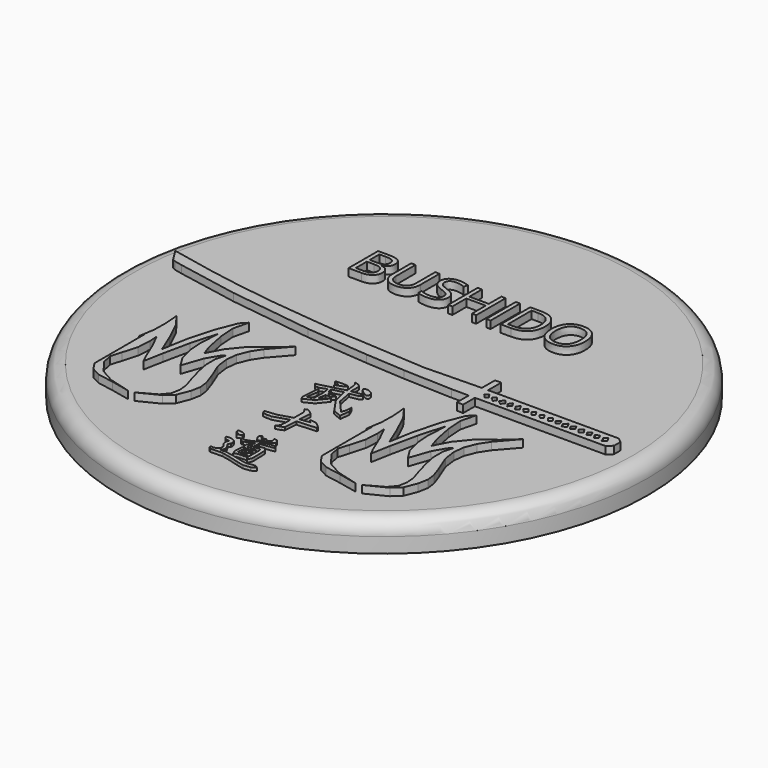
from build123d import *

# Parameters (mm, degrees)
F0_R         = 44.6165868488
F1_DEPTH     = 5.08
F2_R         = 2.54
F3_TEXT_SIZE = 8.7433378212
F4_DEPTH     = 1.27
F6_DEPTH     = 0.508
F8_DEPTH     = 1.27
F12_DEPTH    = 1.27


# Not quite as in the source:
# - Text() gives the source's letters only with a copy of the font that has no kerning and outlines rounded to 1/6400 em; it was checked with that copy


with BuildPart() as f1:
    # F0 (on Top) → F1 (new body)
    with BuildSketch(Plane.XY):
        with Locations((38.1, 0)):
            Circle(F0_R)
    extrude(amount=-F1_DEPTH)

    # F2
    f2_edges = [f1.edges().sort_by_distance(p)[0] for p in [
        (-6.516587, 0, 0),
    ]]
    fillet(f2_edges, radius=F2_R)

    # F3 (on Top) → F4 (join)
    with BuildSketch(Plane.XY):
        with Locations((18.0598776788, 16.4687121287)):
            Text('BUSHIDO', F3_TEXT_SIZE, font='Open Sans', text_align=(TextAlign.LEFT, TextAlign.BOTTOM))
    extrude(amount=F4_DEPTH)

    # F5 (on Top) → F6 (join)
    with BuildSketch(Plane.XY):
        with BuildLine():
            add(Edge.make_bspline(
                [(36.8690937757, -8.8045168668), (36.9262235113, -8.6325223752), (40.9652755864, -8.523144564), (36.521565131, -9.9590094355), (38.386831886, -9.2135998908), (36.830176095, -8.9216822386), (36.8690937757, -8.8045168668)],
                knots=[0, 0, 0, 0, 0.323818666, 0.6224903435, 0.7794095959, 1, 1, 1, 1], degree=3))
        make_face()
        with BuildLine():
            add(Edge.make_bspline(
                [(41.1289557815, -8.1255994737), (41.052845758, -8.4618202993), (42.8844335846, -10.000238978), (42.9689741831, -8.112585225), (41.197261541, -7.8238544756), (41.1289557815, -8.1255994737)],
                knots=[0, 0, 0, 0, 0.3876451352, 0.6521037019, 1, 1, 1, 1], degree=3))
        make_face()
        Polygon((39.8083478212, -7.551421877), (39.1193367541, -7.3983082548), (39.4829809666, -7.9342070967), (39.6935120225, -9.8098535091), (35.9422191978, -10.7859550044), (35.1766496897, -10.9582077712), (35.6551297009, -11.4941066131), (36.4207029343, -11.4941066131), (37.4733582139, -11.0730435699), (37.645611912, -12.2596770525), (37.645611912, -14.173601754), (36.6503708065, -14.556386508), (36.9566008449, -12.8338541836), (36.8226245046, -12.2788157314), (36.4207029343, -11.8194743991), (36.4207029343, -12.3745119199), (36.2527528205, -14.2884366214), (36.2527528205, -14.9953767122), (36.4589802921, -15.4176522046), (38.104955107, -14.6138044074), (39.4829809666, -12.9104116932), (38.8896651566, -13.4080322459), (38.104955107, -13.7716773897), (38.3154861629, -12.6233221963), (39.2150320113, -12.6233221963), (39.5786762238, -12.0108667761), (39.0427783132, -12.0108667761), (38.3537635207, -12.2213987634), (38.3537635207, -11.8768922985), (37.9712446996, -11.4986467292), (37.8296082923, -10.9278071133), (39.712652564, -10.4605872184), (40.3442457318, -13.0061078817), (42.0093610883, -15.4176522046), (43.4830822051, -16.0109698772), (43.6936169863, -14.3267158419), (43.2151332498, -13.2549181581), (43.2151332498, -14.2118800431), (42.8897663951, -15.09228535), (40.9145871592, -12.8176152195), (40.4590815306, -10.3648910299), (41.7988300323, -10.1160807535), (42.3921458423, -9.7907138988), (41.9136658311, -9.427068755), (40.2485504746, -9.7141573206), (40.2485504746, -7.9916249961), align=None)
        Polygon((39.1193367541, -17.3568017781), (38.6665798724, -17.5016503781), (39.1193367541, -18.2741675526), (39.1193367541, -20.3020274639), (36.7674715817, -21.0101678967), (34.7878970206, -21.2193913758), (35.0510981124, -21.753220402), (35.6730744243, -21.8309685588), (36.574345082, -21.8309685588), (39.1006264007, -21.0423562676), (39.1006264007, -22.0924360227), (38.9723666012, -23.1184996665), (38.521733135, -23.5852282494), (39.4069105387, -23.3277231455), (39.8092642426, -23.0863112956), (39.9702042341, -20.8814162761), (43.2695001364, -20.6721927971), (43.2695001364, -20.4307809472), (42.3491622125, -19.6015631681), (41.1289818585, -19.449038431), (41.4846295613, -19.8708384333), (41.6761822999, -19.9479572475), (39.95411098, -20.1893690974), (40.0989577174, -18.0488489568), (39.4835314239, -17.5034259469), align=None)
        Polygon((36.465685972, -27.7904520939), (35.5846919119, -27.6803262532), (35.6803871691, -28.1205289066), (36.2975304264, -28.466149787), (36.1146872415, -28.5084608213), (36.1397303641, -28.7234149873), (36.914074972, -28.4093043748), (36.809604615, -27.9578454792), align=None)
        Polygon((39.1804466829, -27.2458239053), (39.1193367541, -26.9817430526), (38.8000831008, -27.1731354296), (38.8000831008, -27.5463499129), (39.0297546983, -27.9961228371), (39.5869397098, -28.3664732433), (40.0249958038, -27.2784009576), (39.4795276225, -27.6229083538), align=None)
        Polygon((41.3673612083, -26.7059249962), (40.9101359546, -26.6487710178), (40.9225635231, -26.6326684505), (40.8548973501, -26.7138704658), (40.9015711261, -26.9170331416), (40.9766957164, -27.2416770458), (40.0902554393, -28.1890202314), (39.0414074063, -28.9130620658), (38.0263961852, -29.2311012745), (37.4647565186, -29.2311012745), (37.4985933304, -29.4950027019), (37.7286598086, -29.7453738749), (38.1211340427, -29.7859739512), (39.7722199559, -29.1498992592), (38.9661676253, -30.252532206), (39.1075549029, -30.6578476496), (39.0109978616, -31.4302928746), (38.9168218354, -32.5174966777), (39.1666330397, -33.2336314023), (39.5207442189, -33.0261609126), (40.0767624378, -32.9613823011), (40.8199538526, -32.9613823011), (41.1932729185, -32.8749939799), (41.2406399846, -32.766725868), (41.0883910954, -32.4960537255), (40.7293175893, -32.4298856209), (40.0632284582, -32.5840227306), (39.6606065333, -32.5366556644), (39.684291929, -32.4723720551), (39.3933206797, -32.5907878578), (39.4289206542, -31.9954107358), (39.500977844, -31.8164303899), (40.4062718153, -31.8928770721), (40.1003203773, -32.2016964793), (40.1447415352, -32.2630405426), (40.4947884381, -32.0095606148), (41.0145658499, -31.7668251122), (41.1063656211, -31.5388068557), (40.9172587097, -31.3875525708), (40.5635686484, -31.3875525708), (39.875164628, -31.5468534827), (39.4526943564, -31.5508767962), (39.4526943564, -31.0439113528), (39.9654139058, -31.0475337206), (40.07634148, -31.0921929777), (39.8872345686, -31.2531366944), (39.9556346238, -31.3014164567), (40.2260981022, -31.1137784975), (40.7724119723, -30.9232063591), (40.9937053919, -30.7019110769), (40.8166721463, -30.5288992822), (40.5430719256, -30.508780852), (40.0766329326, -30.6154663914), (39.5159046677, -30.6942713389), (39.4848845899, -30.6053459644), (39.3802709877, -30.2150640637), (39.6498478949, -30.0380289555), (40.0692522526, -30.0380289555), (40.7200925539, -30.1231860166), (41.2043756065, -30.0111199484), (41.3665995002, -30.476167798), (41.3665995002, -30.993970111), (41.3665995002, -33.059488982), (41.7219137063, -33.4838654903), (42.0044186505, -32.7821612919), (42.0494154096, -32.4221923947), (41.9654436409, -29.9703944474), (41.5186955414, -29.482565888), (40.7101027668, -29.5962058008), (40.0059856474, -29.8014059663), (40.1065722108, -29.6565592289), (40.1590280235, -28.9832968265), (42.6627248526, -28.631426394), (42.3142741539, -28.2876443354), (42.0158270385, -28.1674900227), (41.2281751633, -28.259254992), (40.1624618085, -28.6310106512), (39.7868566215, -28.5840593278), (40.6597666442, -28.1983558089), (41.70694357, -27.3851653198), (41.6477136314, -27.1292086691), align=None)
        Polygon((35.9769724309, -30.0162881613), (35.522416234, -30.0689209253), (35.5239771307, -30.2073527128), (35.6340296566, -30.4657332599), (35.925898701, -30.7385064662), (36.3089814782, -30.7385064662), (36.5365855396, -30.7726468891), (36.3545045257, -31.2164779752), (36.4569239318, -31.8310111761), (36.9462780654, -32.5252078474), (36.9462780654, -33.0145582557), (36.6048701108, -33.4583893418), (36.0927581787, -33.5494317114), (35.6375463307, -33.4925316274), (35.6375463307, -33.8453166187), (35.9448119998, -34.0615436435), (36.2748429179, -34.0615436435), (37.9705019295, -34.016020596), (39.3019914627, -34.3005284667), (41.1569736898, -34.8012596369), (42.2836206853, -35.0630059838), (43.4785485268, -34.9150635302), (44.229645282, -34.5167554915), (43.7858141959, -34.1867245734), (43.3192253113, -34.1867245734), (42.2608591616, -34.3688093126), (41.1000736058, -34.1412052512), (39.5560152829, -33.7436571717), (38.1062179804, -33.4900617599), (37.1396839619, -33.4900617599), (37.4315604568, -33.2556068897), (37.5272557139, -32.8154042363), (37.4172031879, -32.3752015829), (36.9530729949, -31.6191986203), (37.2210256755, -31.2029216439), (37.2210256755, -30.7627189904), (37.0009243488, -30.375149101), (36.4745929837, -30.0832763314), align=None)
    extrude(amount=F6_DEPTH)

    # F7 (on Top) → F8, piece 2 (join)
    with BuildSketch(Plane.XY):
        Polygon((55.0989850964, -2.054411941), (55.0989850964, 0.7223728814), (55.0989850964, 3.499157238), (54.0519997086, 3.499157238), (54.0519997086, 0.7223728814), (54.0519997086, -2.054411941), (54.0519997086, -4.5237410009), (55.0989850964, -4.5580698874), align=None)
        Polygon((77.1766982581, 0.7223728814), (55.0989850964, 0.7223728814), (55.0989850964, -2.054411941), (77.1766982581, -2.054411941), (77.9960758592, -1.2805538948), (77.9960758592, 0.0850781568), align=None)
        Polygon((55.4676770772, -0.5495769668), (55.9911697711, -0.1171268753), (56.5166056965, -0.8705766641), (56.0507553515, -1.2554092064), align=None, mode=Mode.SUBTRACT)
        Polygon((56.8105473723, -0.6861402884), (57.3112785424, -0.1171268753), (57.8524020593, -0.8637093181), (57.4857708609, -1.2803362069), align=None, mode=Mode.SUBTRACT)
        Polygon((58.1534176673, -0.8227033771), (58.6996718849, -0.1171268753), (59.2185751575, -0.796389675), (58.8066622447, -1.3284424495), align=None, mode=Mode.SUBTRACT)
        Polygon((59.5645725335, -0.7316612404), (59.9970228578, -0.1171268753), (60.3839501347, -0.7544218328), (59.9514998104, -1.3006744206), align=None, mode=Mode.SUBTRACT)
        Polygon((60.8391619827, -0.6406191036), (61.3171316292, -0.1171268753), (61.8392370313, -0.9946705052), (61.2943701054, -1.3461956054), align=None, mode=Mode.SUBTRACT)
        Polygon((62.1137514319, -0.6178585112), (62.6372441258, -0.1171268753), (63.1607368197, -0.8682243291), (62.7261957224, -1.2581418257), align=None, mode=Mode.SUBTRACT)
        Polygon((63.4566254522, -0.5495769668), (63.9573566224, -0.1171268753), (64.3864921622, -0.8452203982), (64.0001298905, -1.1788972485), align=None, mode=Mode.SUBTRACT)
        Polygon((64.8450150694, -0.6406191036), (65.3685077633, -0.1171268753), (65.7781965639, -0.8454637367), (65.3798874015, -1.1754919115), align=None, mode=Mode.SUBTRACT)
        Polygon((66.2106468882, -0.5495769668), (66.7569011058, -0.0716056905), (67.2233903105, -0.7900748888), (66.7689846764, -1.1876788503), align=None, mode=Mode.SUBTRACT)
        Polygon((67.5535171832, -0.5723373264), (68.1680522467, -0.1171268753), (68.4729927468, -0.7814347201), (67.9792940027, -1.1471369255), align=None, mode=Mode.SUBTRACT)
        Polygon((68.805348834, -0.6406191036), (69.3971223737, -0.1171268753), (69.8452441629, -0.9630465539), (69.1695183124, -1.3234347801), align=None, mode=Mode.SUBTRACT)
        Polygon((70.0571767594, -0.5950979188), (70.6944733466, -0.1171268753), (71.0604619573, -0.7871966465), (70.5105653933, -1.1996178642), align=None, mode=Mode.SUBTRACT)
        Polygon((71.4683316256, -0.6406191036), (72.0828629638, -0.1171268753), (72.5076962999, -0.8325627727), (72.0001473271, -1.2649214276), align=None, mode=Mode.SUBTRACT)
        Polygon((72.8339634444, -0.4812951896), (73.4712563063, -0.1171268753), (73.7615411629, -0.8584177471), (73.2247441917, -1.165159686), align=None, mode=Mode.SUBTRACT)
        Polygon((74.1085528936, -0.4812951896), (74.7502955444, -0.1272299119), (75.0751157295, -0.8647188885), (74.4962914293, -1.1840705574), align=None, mode=Mode.SUBTRACT)
        Polygon((75.5264393594, -0.4877723112), (76.0432004537, -0.05083743), (76.4834031071, -0.7781288817), (75.8776194136, -1.2851101326), align=None, mode=Mode.SUBTRACT)
        Polygon((54.0519997086, -2.054411941), (54.0519997086, 0.7223728814), (52.1354645099, -0.3610581856), align=None)
        Polygon((52.1354645099, -0.3610581856), (54.0519997086, 0.7223728814), (44.4104579674, 0.5047083288), (39.4883490074, 0.8158758577), (33.2902302421, 1.207710601), (28.2204418983, 1.5282141745), (22.3446979727, 2.1406705261), (17.3302113618, 2.676569368), (11.0142573323, 3.5569746748), (5.4447322692, 4.5139365599), (-2.0387128387, 6.0450765074), (0.3787099923, 4.8922938064), (4.2831196989, 4.0310281098), (10.042635845, 3.0032707557), (14.7522881235, 2.3467740745), (21.2404921259, 1.6194833212), (25.0300660338, 1.207710601), (28.6202423375, 0.8230696751), (33.0073740295, 0.5457225178), (36.6093113627, 0.3180140399), (45.2411070074, -0.05083743), align=None)
        Polygon((51.1194884385, -2.054411941), (54.0519997086, -2.054411941), (52.1354645099, -0.3610581856), (45.2411070074, -0.05083743), (36.6093113627, 0.3180140399), (33.0073740295, 0.5457225178), (28.6202423375, 0.8230696751), (25.0300660338, 1.207710601), (21.2404921259, 1.6194833212), (14.7522881235, 2.3467740745), (10.042635845, 3.0032707557), (4.2831196989, 4.0310281098), (0.3787099923, 4.8922938064), (-2.0387128387, 6.0450765074), (-0.7181048785, 3.9588990391), (-0.1439258848, 3.6718100079), (1.1766820754, 3.3847214423), (11.4735930766, 1.4516575963), (25.6174996104, -0.4239881176), (36.2015038337, -1.3235330347), (42.8619652595, -1.7445963107), align=None)
    extrude(amount=F8_DEPTH)

    # F10 (on Top) → F12 (join)
    with BuildSketch(Plane.XY):
        Polygon((17.7706117137, -6.5261625266), (18.4039533603, -3.9245185024), (17.4504475065, -4.9308996581), (16.1539996369, -8.2218746236), (14.9249295099, -12.682938627), (14.1510712309, -16.9846784836), (12.7854394122, -13.6616413063), (11.2832459016, -10.4979273445), (9.7127678199, -8.3356775856), (9.9176140829, -10.8165756381), (9.8720947607, -13.3202333516), (9.4624059601, -15.9376949585), (9.7139934405, -15.0523349412), (9.7139934405, -25.6945188614), (10.623191516, -27.0675939089), (12.170908074, -27.8869715101), (14.9021717115, -28.3649411565), (18.1015384634, -29.061992346), (14.4136520429, -28.0592326588), (12.0786624356, -26.7577652401), (10.4135470791, -24.5184727526), (10.0819071327, -22.8507992666), (10.6049413188, -21.0159902042), (11.3322334691, -18.4896100825), (11.4853466256, -16.1929015583), (11.3781978271, -14.6519107457), (12.5427947237, -16.9848664862), (13.820336233, -20.0398896402), (14.3937602257, -21.1885899325), (15.0069678529, -17.877153731), (15.9830684169, -13.3220140404), (16.538106869, -11.2932544715), (17.2469141288, -8.9071343235), (17.0329073771, -12.3905238277), (17.2045830549, -14.8595262412), (17.836754243, -17.2901709146), (18.9659716888, -19.1083994276), (20.1526033087, -15.6633347786), (21.2818207546, -13.7302704668), (21.9516950055, -13.0221188581), (21.4540744527, -14.7446521139), (21.4540744527, -16.8116909033), (21.8399058472, -18.7518696837), (22.4493155583, -21.0031826562), (23.1000492676, -23.0319440878), (23.2531661494, -24.5822217828), (22.9660766526, -26.1133626616), (21.9516950055, -27.3191366858), (19.0405255025, -28.9267474871), (22.4396279039, -27.2299368536), (23.7467720833, -26.0300703118), (24.5753983362, -23.9266396082), (24.8940447672, -22.2651210195), (24.6979864641, -20.7665484912), (24.0089716716, -18.7952049589), (22.9371758505, -16.115709818), (22.6500863536, -14.0103936708), (22.8606174095, -12.1538859374), (23.6070501013, -10.2590999148), (24.6979864641, -8.5939854896), (27.469933997, -5.4124877196), (25.2721654578, -7.4073520071), (22.5352505549, -9.5126690856), (20.5830494269, -11.8859351194), (19.2433009251, -14.4314557827), (18.6308445736, -12.6323659486), (17.9609703227, -9.2638588092), align=None)
        Polygon((57.7353304579, -8.4389333195), (58.3686721045, -5.8372892952), (57.4151662506, -6.843670451), (56.1187183811, -10.1346454165), (54.8896482541, -14.5957094199), (54.1157899751, -18.8974492765), (52.7501581563, -15.5744120992), (51.2479646458, -12.4106981373), (49.6774865641, -10.2484483785), (49.882332827, -12.7293464309), (49.8368135049, -15.2330041445), (49.4271247043, -17.8504657513), (49.6787121846, -16.9651057341), (49.6787121846, -27.6072896542), (50.5879102601, -28.9803647018), (52.1356268181, -29.7997423029), (54.8668904557, -30.2777119494), (58.0662572076, -30.9747631388), (54.3783707871, -29.9720034516), (52.0433811798, -28.6705360329), (50.3782658233, -26.4312435454), (50.0466258769, -24.7635700594), (50.569660063, -22.9287609971), (51.2969522132, -20.4023808754), (51.4500653698, -18.1056723512), (51.3429165712, -16.5646815385), (52.5075134679, -18.8976372791), (53.7850549771, -21.9526604331), (54.3584789698, -23.1013607254), (54.9716865971, -19.7899245239), (55.9477871611, -15.2347848332), (56.5028256132, -13.2060252643), (57.211632873, -10.8199051163), (56.9976261212, -14.3032946205), (57.169301799, -16.772297034), (57.8014729871, -19.2029417074), (58.930690433, -21.0211702204), (60.1173220529, -17.5761055714), (61.2465394987, -15.6430412597), (61.9164137496, -14.934889651), (61.4187931969, -16.6574229068), (61.4187931969, -18.7244616962), (61.8046245914, -20.6646404765), (62.4140343024, -22.915953449), (63.0647680117, -24.9447148806), (63.2178848936, -26.4949925757), (62.9307953967, -28.0261334545), (61.9164137496, -29.2319074786), (59.0052442467, -30.8395182799), (62.404346648, -29.1427076465), (63.7114908274, -27.9428411046), (64.5401170804, -25.839410401), (64.8587635114, -24.1778918124), (64.6627052082, -22.679319284), (63.9736904158, -20.7079757518), (62.9018945946, -18.0284806109), (62.6148050978, -15.9231644637), (62.8253361537, -14.0666567302), (63.5717688455, -12.1718707076), (64.6627052082, -10.5067562825), (67.4346527411, -7.3252585124), (65.2368842019, -9.3201227999), (62.499969299, -11.4254398784), (60.547768171, -13.7987059123), (59.2080196692, -16.3442265755), (58.5955633177, -14.5451367414), (57.9256890668, -11.176629602), align=None)
    extrude(amount=F12_DEPTH)


with BuildPart() as f8:
    # F7 (on Top) → F8 (new body)
    with BuildSketch(Plane.XY):
        Polygon((-64.4438490272, 1.5862523578), (-64.4438490272, 4.3630371802), (-64.4438490272, 7.1398215368), (-65.490834415, 7.1398215368), (-65.490834415, 4.3630371802), (-65.490834415, 1.5862523578), (-65.490834415, -0.8830767021), (-64.4438490272, -0.9174055886), align=None)
        Polygon((-42.3661358654, 4.3630371802), (-64.4438490272, 4.3630371802), (-64.4438490272, 1.5862523578), (-42.3661358654, 1.5862523578), (-41.5467582643, 2.360110404), (-41.5467582643, 3.7257424556), align=None)
        Polygon((-64.0751570463, 3.091087332), (-63.5516643524, 3.5235374235), (-63.026228427, 2.7700876347), (-63.492078772, 2.3852550924), align=None, mode=Mode.SUBTRACT)
        Polygon((-62.7322867513, 2.9545240104), (-62.2315555811, 3.5235374235), (-61.6904320642, 2.7769549807), (-62.0570632626, 2.3603280919), align=None, mode=Mode.SUBTRACT)
        Polygon((-61.3894164562, 2.8179609217), (-60.8431622386, 3.5235374235), (-60.324258966, 2.8442746238), (-60.7361718789, 2.3122218493), align=None, mode=Mode.SUBTRACT)
        Polygon((-59.97826159, 2.9090030584), (-59.5458112657, 3.5235374235), (-59.1588839889, 2.886242466), (-59.5913343132, 2.3399898782), align=None, mode=Mode.SUBTRACT)
        Polygon((-58.7036721408, 3.0000451952), (-58.2257024944, 3.5235374235), (-57.7035970922, 2.6459937936), (-58.2484640181, 2.2944686934), align=None, mode=Mode.SUBTRACT)
        Polygon((-57.4290826917, 3.0228057876), (-56.9055899978, 3.5235374235), (-56.3820973039, 2.7724399697), (-56.8166384012, 2.3825224731), align=None, mode=Mode.SUBTRACT)
        Polygon((-56.0862086713, 3.091087332), (-55.5854775012, 3.5235374235), (-55.1563419614, 2.7954439006), (-55.542704233, 2.4617670503), align=None, mode=Mode.SUBTRACT)
        Polygon((-54.6978190541, 3.0000451952), (-54.1743263602, 3.5235374235), (-53.7646375597, 2.7952005621), (-54.162946722, 2.4651723873), align=None, mode=Mode.SUBTRACT)
        Polygon((-51.9893169403, 3.0683269724), (-51.3747818768, 3.5235374235), (-51.0698413767, 2.8592295787), (-51.5635401209, 2.4935273733), align=None, mode=Mode.SUBTRACT)
        Polygon((-50.7374852896, 3.0000451952), (-50.1457117498, 3.5235374235), (-49.6975899607, 2.6776177449), (-50.3733158112, 2.3172295187), align=None, mode=Mode.SUBTRACT)
        Polygon((-49.4856573641, 3.04556638), (-48.8483607769, 3.5235374235), (-48.4823721662, 2.8534676523), (-49.0322687302, 2.4410464346), align=None, mode=Mode.SUBTRACT)
        Polygon((-48.0745024979, 3.0000451952), (-47.4599711597, 3.5235374235), (-47.0351378236, 2.8081015261), (-47.5426867965, 2.3757428712), align=None, mode=Mode.SUBTRACT)
        Polygon((-53.3321872354, 3.091087332), (-52.7859330177, 3.5690586083), (-52.319443813, 2.85058941), (-52.7738494472, 2.4529854485), align=None, mode=Mode.SUBTRACT)
        Polygon((-46.7088706791, 3.1593691092), (-46.0715778172, 3.5235374235), (-45.7812929606, 2.7822465517), (-46.3180899318, 2.4755046128), align=None, mode=Mode.SUBTRACT)
        Polygon((-45.43428123, 3.1593691092), (-44.7925385792, 3.5134343869), (-44.467718394, 2.7759454103), (-45.0465426942, 2.4565937414), align=None, mode=Mode.SUBTRACT)
        Polygon((-44.0163947642, 3.1528919876), (-43.4996336699, 3.5898268688), (-43.0594310164, 2.8625354171), (-43.6652147099, 2.3555541662), align=None, mode=Mode.SUBTRACT)
        Polygon((-65.490834415, 1.5862523578), (-65.490834415, 4.3630371802), (-67.4073696136, 3.2796061132), align=None)
        Polygon((-67.4073696136, 3.2796061132), (-65.490834415, 4.3630371802), (-75.1323761561, 4.1453726276), (-80.0544851161, 4.4565401565), (-86.2526038814, 4.8483748998), (-91.3223922253, 5.1688784733), (-97.1981361508, 5.7813348249), (-102.2126227617, 6.3172336668), (-108.5285767913, 7.1976389736), (-114.0981018543, 8.1546008587), (-121.5815469623, 9.6857408062), (-119.1641241312, 8.5329581052), (-115.2597144246, 7.6716924086), (-109.5001982785, 6.6439350545), (-104.790546, 5.9874383733), (-98.3023419976, 5.26014762), (-94.5127680898, 4.8483748998), (-90.9225917861, 4.4637339739), (-86.535460094, 4.1863868166), (-82.9335227609, 3.9586783387), (-74.3017271161, 3.5898268688), align=None)
        Polygon((-68.423345685, 1.5862523578), (-65.490834415, 1.5862523578), (-67.4073696136, 3.2796061132), (-74.3017271161, 3.5898268688), (-82.9335227609, 3.9586783387), (-86.535460094, 4.1863868166), (-90.9225917861, 4.4637339739), (-94.5127680898, 4.8483748998), (-98.3023419976, 5.26014762), (-104.790546, 5.9874383733), (-109.5001982785, 6.6439350545), (-115.2597144246, 7.6716924086), (-119.1641241312, 8.5329581052), (-121.5815469623, 9.6857408062), (-120.260939002, 7.5995633379), (-119.6867600083, 7.3124743067), (-118.3661520481, 7.0253857411), (-108.0692410469, 5.0923218951), (-93.9253345132, 3.2166761812), (-83.3413302898, 2.3171312641), (-76.6808688641, 1.8960679881), align=None)
    extrude(amount=F8_DEPTH)


solid = f1.part
